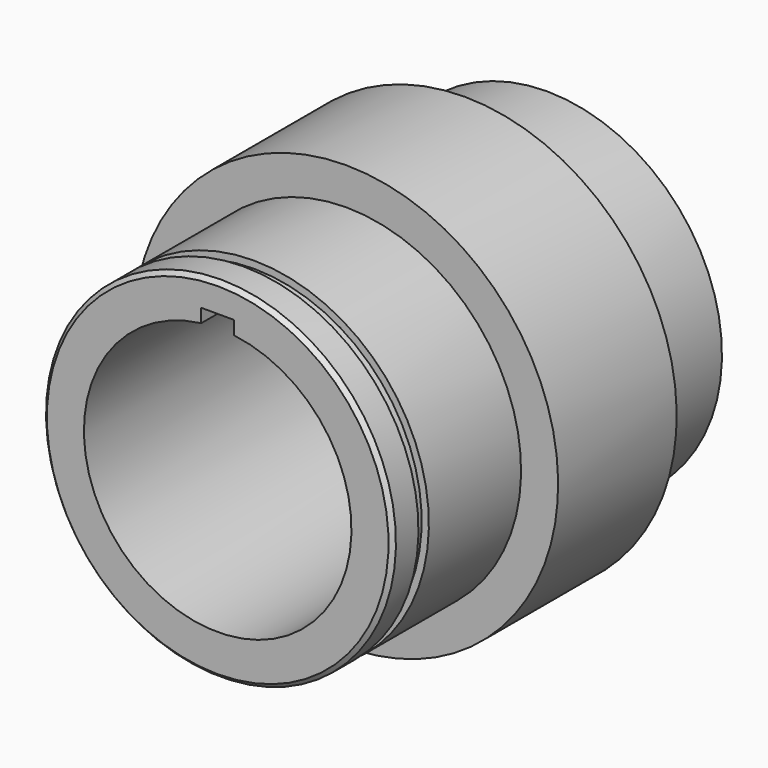
from build123d import *

# Parameters (mm, degrees)
F4_DEPTH = 100.001
F5_SIZE  = 1


with BuildPart() as f1:
    # F0 (on Right) → F1 (revolve)
    with BuildSketch(Plane.YZ):
        Polygon((-142.5, 42.5), (-142.5, 0), (-42.5, 0), (-42.5, 42.5), (-67.5, 42.5), (-67.5, 51.5), (-103.5, 51.5), (-103.5, 42.5), (-131.5, 42.5), (-131.5, 40.75), (-134.65, 40.75), (-134.65, 42.5), align=None)
    revolve(axis=Axis((0, -92.5, 0), (0, -1, 0)))

    # F3 (on face) → F4 (cut, through all)
    with BuildSketch(Plane.XZ.offset(142.5)):
        with BuildLine():
            Line((-4, 35.5529068457), (-4, 32.2529068457))
            ThreePointArc((-4, 32.2529068457), (0, -32.5), (4, 32.2529068457))
            Line((4, 32.2529068457), (4, 35.5529068457))
            Line((4, 35.5529068457), (-4, 35.5529068457))
        make_face()
    extrude(amount=-F4_DEPTH, mode=Mode.SUBTRACT)

    # F5
    f5_edges = [f1.edges().sort_by_distance(p)[0] for p in [
        (0, -142.5, -42.5),
        (0, -42.5, -32.5),
    ]]
    chamfer(f5_edges, length=F5_SIZE)


solid = f1.part
